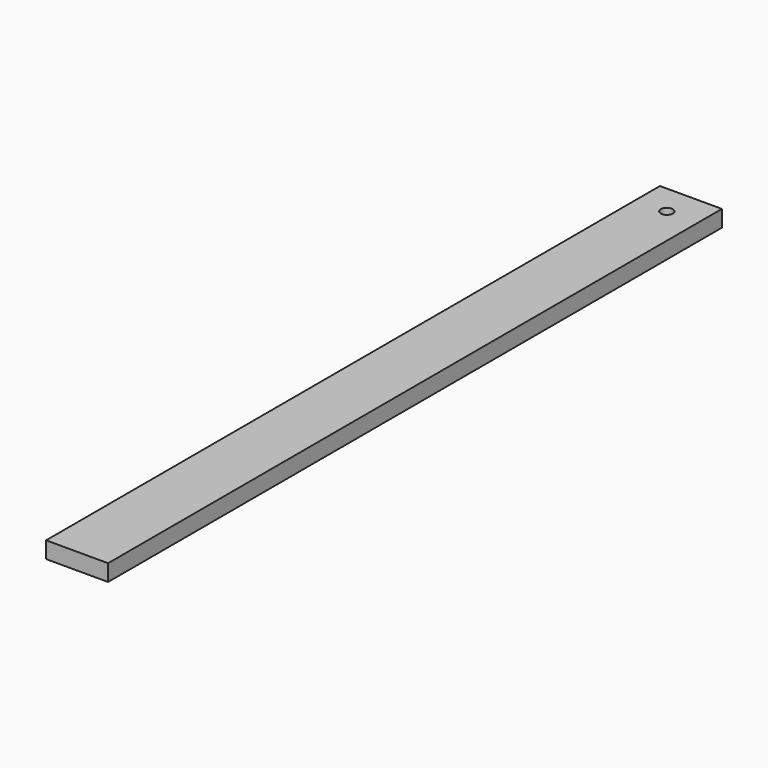
from build123d import *

# Parameters (mm, degrees)
F0_W     = 26.162
F0_H     = 12.7
F1_DEPTH = 6.985


with BuildPart() as f1:
    # F0 (on Top) → F1 (new body)
    with BuildSketch(Plane.XY):
        with BuildLine():
            Line((13.081, -149.225), (13.081, 149.225))
            Line((13.081, 149.225), (2.54, 149.225))
            ThreePointArc((2.54, 149.225), (0, 146.685), (-2.54, 149.225))
            Line((-2.54, 149.225), (-13.081, 149.225))
            Line((-13.081, 149.225), (-13.081, -149.225))
            Line((-13.081, -149.225), (13.081, -149.225))
        make_face()
        with BuildLine():
            Line((2.54, 149.225), (13.081, 149.225))
            Line((13.081, 149.225), (13.081, 161.925))
            Line((13.081, 161.925), (-13.081, 161.925))
            Line((-13.081, 161.925), (-13.081, 149.225))
            Line((-13.081, 149.225), (-2.54, 149.225))
            ThreePointArc((-2.54, 149.225), (0, 151.765), (2.54, 149.225))
        make_face()
        with Locations((0, -155.575)):
            Rectangle(F0_W, F0_H)
    extrude(amount=F1_DEPTH)


solid = f1.part
